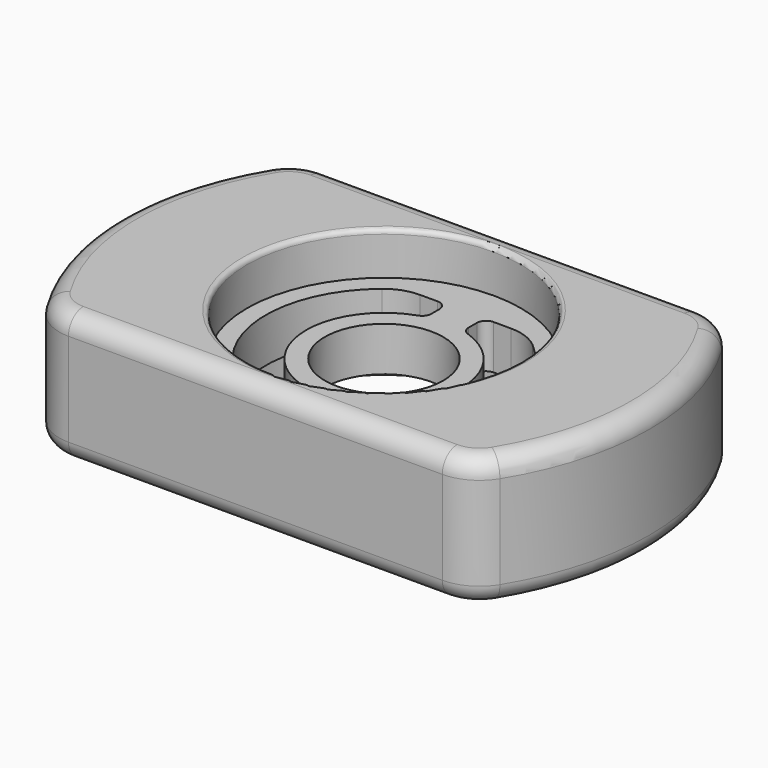
from build123d import *

# Parameters (mm, degrees)
F3_DEPTH      = 12.5
F5_DEPTH      = 25
F6_R          = 5
F6_2_R        = 5
F7_F1_R       = 1
F7_F2_R       = 1
F7_F3_R       = 1
F7_F4_R       = 1
F7_F5_R       = 1
F7_F6_R       = 1
F7_F7_R       = 1
F7_F8_R       = 1
F7_2_T1_DEPTH = 4.7461491674
F7_2_T3_DEPTH = 6.508829184
F8_R          = 5
F9_R          = 2
F10_R         = 1
F11_R         = 0.5
F12_R         = 0.99999
F13_R         = 0.5


# Not quite as in the source:
# - a fillet or chamfer that OpenCascade refuses, or shapes differently, is made with other operations: its cross-section is extruded or revolved along the edge and cut away or added
# - a fillet or chamfer is up to 0.001 mm smaller than in the source, because OpenCascade refuses the exact size


with BuildPart() as f1:
    # F0 (on Front) → F1 (revolve)
    with BuildSketch(Plane.XZ):
        Polygon((6.35, 4.7625), (6.35, 0), (12.7, 0), (14.7, 0), (14.7, -1.5), (14.7, -4.61875), (24.5, -4.61875), (28.5, -4.61875), (28.5, 2.38125), (28.5, 9.38125), (24.5, 9.38125), (14.7, 9.38125), (14.7, 6.2625), (14.7, 4.7625), (12.7, 4.7625), align=None)
    revolve(axis=Axis((0, 0, 2.38125), (0, 0, 1)))

    # F2 (on Top) → F3 (cut, symmetric)
    with BuildSketch(Plane.XY):
        Polygon((43.4596711934, -17.25), (17.25, -17.25), (-17.25, -17.25), (-37.0058989125, -17.25), (-37.0058989125, -42.7323755096), (43.4596711934, -42.7323755096), align=None)
        Polygon((-17.25, 17.25), (17.25, 17.25), (41.6040706777, 17.25), (41.6040706777, 42.1191624585), (-37.1745894389, 42.1191624585), (-37.1745894389, 17.25), align=None)
    extrude(amount=F3_DEPTH, both=True, mode=Mode.SUBTRACT)


with BuildPart() as f1b:
    # F0 (on Front) → F1, piece 2 (revolve)
    with BuildSketch(Plane.XZ):
        with BuildLine():
            Line((13.7, -0.7476008326), (12.7, -0.7476008326))
            Line((12.7, -0.7476008326), (0, -0.7476008326))
            Line((0, -0.7476008326), (0, -3.9319758326))
            ThreePointArc((0, -3.9319758326), (4.3942490964, -4.3344919718), (8.6518969432, -5.49375))
            Line((8.6518969432, -5.49375), (10.5085438117, -5.49375))
            Line((10.5085438117, -5.49375), (13.7, -5.49375))
            Line((13.7, -5.49375), (13.7, -1.5))
            Line((13.7, -1.5), (13.7, -0.7476008326))
        make_face()
    revolve(axis=Axis((0, 0, 2.38125), (0, 0, 1)))


with BuildPart() as f1c:
    # F0 (on Front) → F1, piece 3 (revolve)
    with BuildSketch(Plane.XZ):
        with BuildLine():
            Line((0, 8.6944758326), (0, 6.2577016652))
            Line((0, 6.2577016652), (0, 5.5101008326))
            Line((0, 5.5101008326), (12.7, 5.5101008326))
            Line((12.7, 5.5101008326), (13.7, 5.5101008326))
            Line((13.7, 5.5101008326), (13.7, 6.2625))
            Line((13.7, 6.2625), (13.7, 10.25625))
            Line((13.7, 10.25625), (10.5085438117, 10.25625))
            Line((10.5085438117, 10.25625), (8.6518969432, 10.25625))
            ThreePointArc((8.6518969432, 10.25625), (4.3942490964, 9.0969919718), (0, 8.6944758326))
        make_face()
    revolve(axis=Axis((0, 0, 2.38125), (0, 0, 1)))

    # F10
    f10_edges = [f1c.edges().sort_by_distance(p)[0] for p in [
        (-13.7, 0, 10.25625),
    ]]
    fillet(f10_edges, radius=F10_R)


with BuildPart() as f5_tool:
    # F4 (on face) → F5 (new body)
    with BuildSketch(Plane.XY.offset(4.7625)):
        with BuildLine():
            ThreePointArc((-6.4411438468, 10.9453947368), (-12.7, 0), (-6.4411438468, -10.9453947368))
            Line((-6.4411438468, -10.9453947368), (-2, -10.9453947368))
            Line((-2, -10.9453947368), (-2, -8.1069414701))
            ThreePointArc((-2, -8.1069414701), (-8.35, 0), (-2, 8.1069414701))
            Line((-2, 8.1069414701), (-2, 10.9453947368))
            Line((-2, 10.9453947368), (-6.4411438468, 10.9453947368))
        make_face()
        with BuildLine():
            Line((2, -10.9453947368), (6.4411438468, -10.9453947368))
            ThreePointArc((6.4411438468, -10.9453947368), (12.7, 0), (6.4411438468, 10.9453947368))
            Line((6.4411438468, 10.9453947368), (2, 10.9453947368))
            Line((2, 10.9453947368), (2, 8.1069414701))
            ThreePointArc((2, 8.1069414701), (8.35, 0), (2, -8.1069414701))
            Line((2, -8.1069414701), (2, -10.9453947368))
        make_face()
    extrude(amount=-F5_DEPTH)


with BuildPart() as f1_1:
    add(f1.part)

    # F5: cut by f5_tool
    add(f5_tool.part, mode=Mode.SUBTRACT)

    # F6
    f6_edges = [f1_1.edges().sort_by_distance(p)[0] for p in [
        (6.441144, 10.945395, 2.38125),
        (-6.441144, 10.945395, 2.38125),
        (-6.441144, -10.945395, 2.38125),
        (6.441144, -10.945395, 2.38125),
    ]]
    fillet(f6_edges, radius=F6_R)

    # F7: fillet of radius 1 on 8 edges, made by hand

    # F7_f1
    f7_f1_edges = [f1_1.edges().sort_by_distance(p)[0] for p in [
        (-2, 10.9453947368, 2.38125),
    ]]
    fillet(f7_f1_edges, radius=F7_F1_R)

    # F7_f2
    f7_f2_edges = [f1_1.edges().sort_by_distance(p)[0] for p in [
        (-2, 8.1069414701, 2.38125),
    ]]
    fillet(f7_f2_edges, radius=F7_F2_R)

    # F7_f3
    f7_f3_edges = [f1_1.edges().sort_by_distance(p)[0] for p in [
        (-2, -8.1069414701, 2.38125),
    ]]
    fillet(f7_f3_edges, radius=F7_F3_R)

    # F7_f4
    f7_f4_edges = [f1_1.edges().sort_by_distance(p)[0] for p in [
        (-2, -10.9453947368, 2.38125),
    ]]
    fillet(f7_f4_edges, radius=F7_F4_R)

    # F7_f5
    f7_f5_edges = [f1_1.edges().sort_by_distance(p)[0] for p in [
        (2, -10.9453947368, 2.38125),
    ]]
    fillet(f7_f5_edges, radius=F7_F5_R)

    # F7_f6
    f7_f6_edges = [f1_1.edges().sort_by_distance(p)[0] for p in [
        (2, -8.1069414701, 2.38125),
    ]]
    fillet(f7_f6_edges, radius=F7_F6_R)

    # F7_f7
    f7_f7_edges = [f1_1.edges().sort_by_distance(p)[0] for p in [
        (2, 8.1069414701, 2.38125),
    ]]
    fillet(f7_f7_edges, radius=F7_F7_R)

    # F7_f8
    f7_f8_edges = [f1_1.edges().sort_by_distance(p)[0] for p in [
        (2, 10.9453947368, 2.38125),
    ]]
    fillet(f7_f8_edges, radius=F7_F8_R)

    # F8
    f8_edges = [f1_1.edges().sort_by_distance(p)[0] for p in [
        (-22.686725, -17.25, 2.38125),
        (22.686725, -17.25, 2.38125),
        (-22.686725, 17.25, 2.38125),
        (22.686725, 17.25, 2.38125),
    ]]
    fillet(f8_edges, radius=F8_R)

    # F9
    f9_edges = [f1_1.edges().sort_by_distance(p)[0] for p in [
        (0, 17.25, 9.38125),
        (0, 17.25, -4.61875),
    ]]
    fillet(f9_edges, radius=F9_R)

    # F11
    f11_edges = [f1_1.edges().sort_by_distance(p)[0] for p in [
        (-14.7, 0, 9.38125),
    ]]
    fillet(f11_edges, radius=F11_R)

    # F13
    f13_edges = [f1_1.edges().sort_by_distance(p)[0] for p in [
        (-14.7, 0, -4.61875),
    ]]
    fillet(f13_edges, radius=F13_R)


with BuildPart() as f1b_1:
    add(f1b.part)

    # F5: cut by f5_tool
    add(f5_tool.part, mode=Mode.SUBTRACT)

    # F6#2
    f6_2_edges = [f1b_1.edges().sort_by_distance(p)[0] for p in [
        (6.441144, 10.945395, -3.120675),
        (-6.441144, 10.945395, -3.120675),
        (-6.441144, -10.945395, -3.120675),
        (6.441144, -10.945395, -3.120675),
    ]]
    fillet(f6_2_edges, radius=F6_2_R)

    # F7#2: fillet of radius 1 on 8 edges, made by hand

    # F7_2_s2 → F7_2_t1 (join)
    with BuildSketch(Plane.XY.offset(-5.49375)):
        with BuildLine():
            ThreePointArc((-3, 10.9453947368), (-2.2928932188, 10.652501518), (-2, 9.9453947368))
            Line((-2, 9.9453947368), (-1.98, 9.9453947368))
            Line((-1.98, 9.9453947368), (-1.98, 10.9653947368))
            Line((-1.98, 10.9653947368), (-3, 10.9653947368))
            Line((-3, 10.9653947368), (-3, 10.9453947368))
        make_face()
        with BuildLine():
            ThreePointArc((3, -10.9453947368), (2.2928932188, -10.652501518), (2, -9.9453947368))
            Line((2, -9.9453947368), (1.98, -9.9453947368))
            Line((1.98, -9.9453947368), (1.98, -10.9653947368))
            Line((1.98, -10.9653947368), (3, -10.9653947368))
            Line((3, -10.9653947368), (3, -10.9453947368))
        make_face()
        with BuildLine():
            ThreePointArc((2, 9.9453947368), (2.2928932188, 10.652501518), (3, 10.9453947368))
            Line((3, 10.9453947368), (3, 10.9653947368))
            Line((3, 10.9653947368), (1.98, 10.9653947368))
            Line((1.98, 10.9653947368), (1.98, 9.9453947368))
            Line((1.98, 9.9453947368), (2, 9.9453947368))
        make_face()
        with BuildLine():
            ThreePointArc((-2, -9.9453947368), (-2.2928932188, -10.652501518), (-3, -10.9453947368))
            Line((-3, -10.9453947368), (-3, -10.9653947368))
            Line((-3, -10.9653947368), (-1.98, -10.9653947368))
            Line((-1.98, -10.9653947368), (-1.98, -9.9453947368))
            Line((-1.98, -9.9453947368), (-2, -9.9453947368))
        make_face()
    extrude(amount=F7_2_T1_DEPTH)

    # F7_2_s4 → F7_2_t3 (join)
    with BuildSketch(Plane.XY.offset(-7.2564300165)):
        with BuildLine():
            ThreePointArc((2.679144385, 7.908519796), (2.1873329049, 8.2729196832), (2, 8.8556479153))
            Line((2, 8.8556479153), (1.98, 8.8556479153))
            Line((1.98, 8.8556479153), (1.98, 8.1069414701))
            Line((1.98, 8.1069414701), (1.9952095808, 8.0875236462))
            ThreePointArc((1.9952095808, 8.0875236462), (2.3360659907, 7.9957298408), (2.6727272727, 7.8895772336))
            Line((2.6727272727, 7.8895772336), (2.679144385, 7.908519796))
        make_face()
        with BuildLine():
            ThreePointArc((-2, 8.8556479153), (-2.1873329049, 8.2729196832), (-2.679144385, 7.908519796))
            Line((-2.679144385, 7.908519796), (-2.6727272727, 7.8895772336))
            ThreePointArc((-2.6727272727, 7.8895772336), (-2.3360659907, 7.9957298408), (-1.9952095808, 8.0875236462))
            Line((-1.9952095808, 8.0875236462), (-1.98, 8.1069414701))
            Line((-1.98, 8.1069414701), (-1.98, 8.8556479153))
            Line((-1.98, 8.8556479153), (-2, 8.8556479153))
        make_face()
        with BuildLine():
            ThreePointArc((2, -8.8556479153), (2.1873329049, -8.2729196832), (2.679144385, -7.908519796))
            Line((2.679144385, -7.908519796), (2.6727272727, -7.8895772336))
            ThreePointArc((2.6727272727, -7.8895772336), (2.3360659907, -7.9957298408), (1.9952095808, -8.0875236462))
            Line((1.9952095808, -8.0875236462), (1.98, -8.1069414701))
            Line((1.98, -8.1069414701), (1.98, -8.8556479153))
            Line((1.98, -8.8556479153), (2, -8.8556479153))
        make_face()
        with BuildLine():
            ThreePointArc((-2.679144385, -7.908519796), (-2.1873329049, -8.2729196832), (-2, -8.8556479153))
            Line((-2, -8.8556479153), (-1.98, -8.8556479153))
            Line((-1.98, -8.8556479153), (-1.98, -8.1069414701))
            Line((-1.98, -8.1069414701), (-1.9952095808, -8.0875236462))
            ThreePointArc((-1.9952095808, -8.0875236462), (-2.3360659907, -7.9957298408), (-2.6727272727, -7.8895772336))
            Line((-2.6727272727, -7.8895772336), (-2.679144385, -7.908519796))
        make_face()
    extrude(amount=F7_2_T3_DEPTH)

    # F12 (radius 1 in the source; OpenCascade refuses exactly that, so slightly less here)
    f12_edges = [f1b_1.edges().sort_by_distance(p)[0] for p in [
        (-13.7, 0, -5.49375),
    ]]
    fillet(f12_edges, radius=F12_R)


solid = f1_1.part
